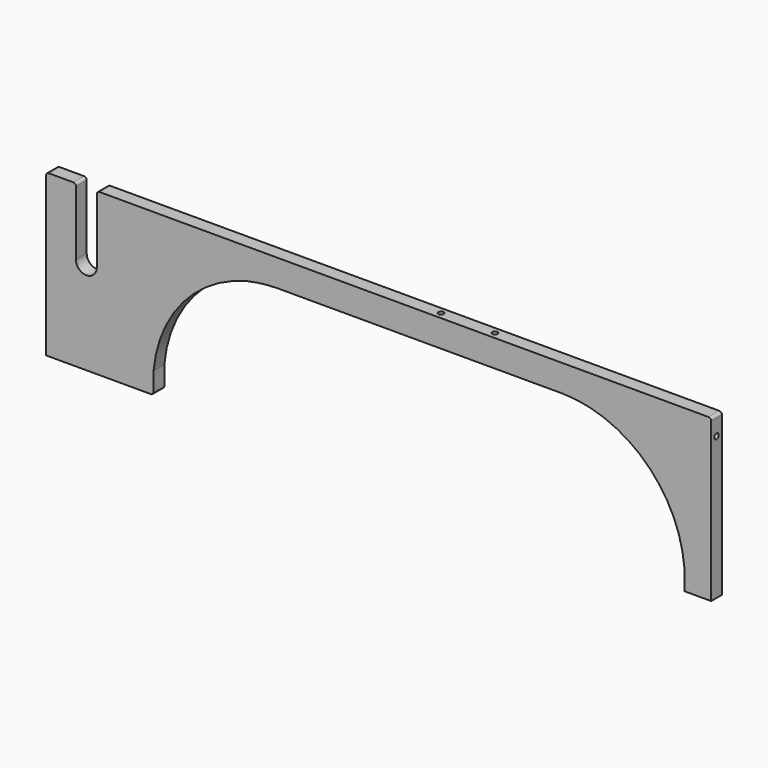
from build123d import *

# Parameters (mm, degrees)
F1_DEPTH    = 5
F2_T1_DEPTH = 10
F2_T3_DEPTH = 20
F4_R        = 2
F5_DEPTH    = 10
F6_R        = 2
F7_DEPTH    = 10
F8_R        = 2
F9_DEPTH    = 10


# Not quite as in the source:
# - a fillet or chamfer that OpenCascade refuses, or shapes differently, is made with other operations: its cross-section is extruded or revolved along the edge and cut away or added
# - two fillets or chamfers of one size are made in one step


with BuildPart() as f1:
    # F0 (on Front) → F1 (new body, symmetric)
    with BuildSketch(Plane.XZ):
        with BuildLine():
            Line((-277.5, 60), (-277.5, -60))
            Line((-277.5, -60), (-197.5, -60))
            Line((-197.5, -60), (-197.5, -44.1662961254))
            ThreePointArc((-197.5, -44.1662961254), (-175.6633710032, 7.8544741443), (-127.5852874265, 37.3755985301))
            ThreePointArc((-127.5852874265, 37.3755985301), (-116.7403394644, 39.2599448569), (-105.7578089833, 40))
            Line((-105.7578089833, 40), (105.7578089833, 40))
            ThreePointArc((105.7578089833, 40), (116.7403394644, 39.2599448569), (127.5852874265, 37.3755985301))
            ThreePointArc((127.5852874265, 37.3755985301), (175.6633710032, 7.8544741443), (197.5, -44.1662961254))
            Line((197.5, -44.1662961254), (197.5, -60))
            Line((197.5, -60), (217.5, -60))
            Line((217.5, -60), (217.5, 40))
            Line((217.5, 40), (217.5, 60))
            Line((217.5, 60), (-239.75, 60))
            Line((-239.75, 60), (-239.75, 10))
            ThreePointArc((-239.75, 10), (-247.5, 2.25), (-255.25, 10))
            Line((-255.25, 10), (-255.25, 60))
            Line((-255.25, 60), (-277.5, 60))
        make_face()
    extrude(amount=F1_DEPTH, both=True)

    # F2: fillet of radius 2 on 6 edges, made by hand

    # F2_s2 → F2_t1 (join)
    with BuildSketch(Plane.XZ.offset(-5)):
        with BuildLine():
            ThreePointArc((-197.4924301703, -44.0790595559), (-197.4981066464, -44.1658995935), (-197.5, -44.252904362))
            Line((-197.5, -44.252904362), (-197.5, -44.1662961254))
            ThreePointArc((-197.5, -44.1662961254), (-197.4962254546, -44.1226769409), (-197.4924301703, -44.0790595559))
        make_face()
    extrude(amount=F2_T1_DEPTH)

    # F2_s4 → F2_t3 (cut)
    with BuildSketch(Plane.XZ.offset(-10)):
        with BuildLine():
            ThreePointArc((-255.25, 58), (-255.8357864376, 59.4142135624), (-257.25, 60))
            Line((-257.25, 60), (-255.25, 60))
            Line((-255.25, 60), (-255.25, 58))
        make_face()
        with BuildLine():
            ThreePointArc((-275.5, 60), (-276.9142135624, 59.4142135624), (-277.5, 58))
            Line((-277.5, 58), (-277.5, 60))
            Line((-277.5, 60), (-275.5, 60))
        make_face()
        with BuildLine():
            ThreePointArc((-199.5, -60), (-198.0857864376, -59.4142135624), (-197.5, -58))
            Line((-197.5, -58), (-197.5, -60))
            Line((-197.5, -60), (-199.5, -60))
        make_face()
        with BuildLine():
            ThreePointArc((-237.75, 60), (-239.1642135624, 59.4142135624), (-239.75, 58))
            Line((-239.75, 58), (-239.75, 60))
            Line((-239.75, 60), (-237.75, 60))
        make_face()
        with BuildLine():
            ThreePointArc((217.5, 58), (216.9142135624, 59.4142135624), (215.5, 60))
            Line((215.5, 60), (217.5, 60))
            Line((217.5, 60), (217.5, 58))
        make_face()
    extrude(amount=F2_T3_DEPTH, mode=Mode.SUBTRACT)

    # F4 (on face) → F5 (cut)
    with BuildSketch(Plane.XY.offset(60)):
        with Locations((12.5, 0)):
            Circle(F4_R)
        with Locations((52.5, 0)):
            Circle(F4_R)
    extrude(amount=-F5_DEPTH, mode=Mode.SUBTRACT)

    # F6 (on face) → F7 (cut)
    with BuildSketch(Plane.YZ.offset(217.5)):
        with Locations((0, 46)):
            Circle(F6_R)
    extrude(amount=-F7_DEPTH, mode=Mode.SUBTRACT)

    # F8 (on face) → F9 (cut)
    with BuildSketch(Plane(origin=(-277.5, 0, 0), x_dir=(0, -1, 0), z_dir=(-1, 0, 0))):
        with Locations((0, 50)):
            Circle(F8_R)
    extrude(amount=-F9_DEPTH, mode=Mode.SUBTRACT)


solid = f1.part
